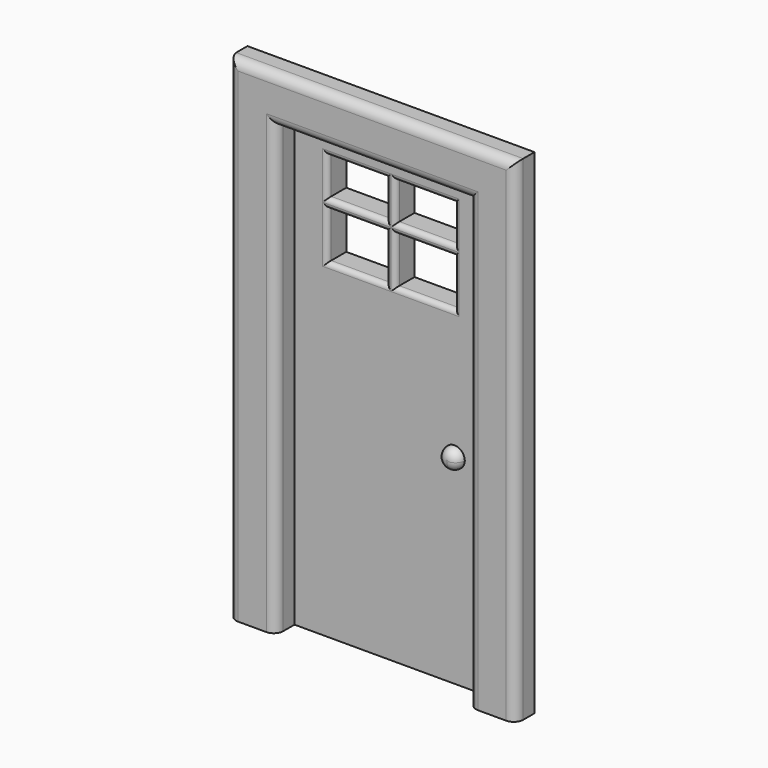
from build123d import *

# Parameters (mm, degrees)
F1_DEPTH  = 2.54
F0_W      = 0.508
F0_H      = 0.508
F0_H_2    = 2.032
F0_W_2    = 3.175
F0_H_3    = 2.54
F2_DEPTH  = 1.27
F3_DEPTH  = 1.778
F4_R      = 0.50799
F5_R      = 0.25399
F6_W      = 1.27
F6_H      = 25.4
F7_DEPTH  = 1.27
F8_W      = 1.27
F8_H      = 25.4
F9_DEPTH  = 1.27
F11_DEPTH = 1.27
F12_R     = 0.508


# Not quite as in the source:
# - a fillet or chamfer is up to 0.001 mm smaller than in the source, because OpenCascade refuses the exact size


with BuildPart() as f1:
    # F0 (on Front) → F1 (new body)
    with BuildSketch(Plane.XZ):
        Polygon((0, 24.13), (0, 0), (1.27, 0), (1.27, 25.4), (-11.684, 25.4), (-11.684, 0), (-10.414, 0), (-10.414, 24.13), align=None)
    extrude(amount=F1_DEPTH)

    # F0 (on Front) → F2 (join)
    with BuildSketch(Plane.XZ):
        Polygon((-1.778, 0), (0, 0), (0, 24.13), (-10.414, 24.13), (-10.414, 0), align=None)
        with BuildLine():
            ThreePointArc((-1.2223680419, 10.7806390151), (-1.3851088746, 10.3877478897), (-1.778, 10.2250070571))
            ThreePointArc((-1.778, 10.2250070571), (-2.1708911254, 11.1735301405), (-1.2223680419, 10.7806390151))
        make_face(mode=Mode.SUBTRACT)
        Polygon((-4.953, 22.86), (-1.778, 22.86), (-1.778, 20.828), (-1.778, 20.32), (-1.778, 17.78), (-4.953, 17.78), (-5.461, 17.78), (-8.636, 17.78), (-8.636, 20.32), (-8.636, 20.828), (-8.636, 22.86), (-5.461, 22.86), align=None, mode=Mode.SUBTRACT)
        with Locations((-5.207, 20.574)):
            Rectangle(F0_W, F0_H)
        with Locations((-5.207, 21.844)):
            Rectangle(F0_W, F0_H_2)
        with Locations((-7.0485, 20.574)):
            Rectangle(F0_W_2, F0_H)
        with Locations((-5.207, 19.05)):
            Rectangle(F0_W, F0_H_3)
        with Locations((-3.3655, 20.574)):
            Rectangle(F0_W_2, F0_H)
        with BuildLine():
            ThreePointArc((-1.2223680419, 10.7806390151), (-2.1708911254, 11.1735301405), (-1.778, 10.2250070571))
            ThreePointArc((-1.778, 10.2250070571), (-1.3851088746, 10.3877478897), (-1.2223680419, 10.7806390151))
        make_face()
    extrude(amount=F2_DEPTH)

    # F0 (on Front) → F3 (join)
    with BuildSketch(Plane.XZ):
        with BuildLine():
            ThreePointArc((-1.2223680419, 10.7806390151), (-2.1708911254, 11.1735301405), (-1.778, 10.2250070571))
            ThreePointArc((-1.778, 10.2250070571), (-1.3851088746, 10.3877478897), (-1.2223680419, 10.7806390151))
        make_face()
    extrude(amount=F3_DEPTH)

    # F4 (radius 0.508 in the source; OpenCascade refuses exactly that, so slightly less here)
    f4_edges = [f1.edges().sort_by_distance(p)[0] for p in [
        (-10.414, -2.54, 12.065),
        (0, -2.54, 12.065),
        (-5.207, -2.54, 24.13),
        (-1.778, -1.778, 11.336271),
    ]]
    fillet(f4_edges, radius=F4_R)

    # F5 (radius 0.254 in the source; OpenCascade refuses exactly that, so slightly less here)
    f5_edges = [f1.edges().sort_by_distance(p)[0] for p in [
        (-3.3655, -1.27, 22.86),
        (-1.778, -1.27, 21.844),
        (-3.3655, -1.27, 20.828),
        (-1.778, -1.27, 19.05),
        (-3.3655, -1.27, 17.78),
        (-7.0485, -1.27, 17.78),
        (-5.461, -1.27, 19.05),
        (-7.0485, -1.27, 22.86),
        (-8.636, -1.27, 21.844),
        (-8.636, -1.27, 19.05),
        (-7.0485, -1.27, 20.32),
        (-4.953, -1.27, 21.844),
        (-7.0485, -1.27, 20.828),
        (-5.461, -1.27, 21.844),
        (-4.953, -1.27, 19.05),
        (-3.3655, -1.27, 20.32),
    ]]
    fillet(f5_edges, radius=F5_R)

    # F6 (on face) → F7 (join)
    with BuildSketch(Plane.YZ.offset(1.27)):
        with Locations((-1.905, 12.7)):
            Rectangle(F6_W, F6_H)
    extrude(amount=F7_DEPTH)

    # F8 (on face) → F9 (join)
    with BuildSketch(Plane(origin=(-11.684, 0, 0), x_dir=(0, -1, 0), z_dir=(-1, 0, 0))):
        with Locations((1.905, 12.7)):
            Rectangle(F8_W, F8_H)
    extrude(amount=F9_DEPTH)

    # F10 (on face) → F11 (join)
    with BuildSketch(Plane.XY.offset(25.4)):
        Polygon((-12.954, -1.27), (-12.954, -2.54), (2.54, -2.54), (2.54, -1.27), (1.27, -1.27), (-11.684, -1.27), align=None)
    extrude(amount=F11_DEPTH)

    # F12
    f12_edges = [f1.edges().sort_by_distance(p)[0] for p in [
        (-12.954, -2.54, 13.335),
        (-5.207, -2.54, 26.67),
        (2.54, -2.54, 13.335),
    ]]
    fillet(f12_edges, radius=F12_R)


solid = f1.part
